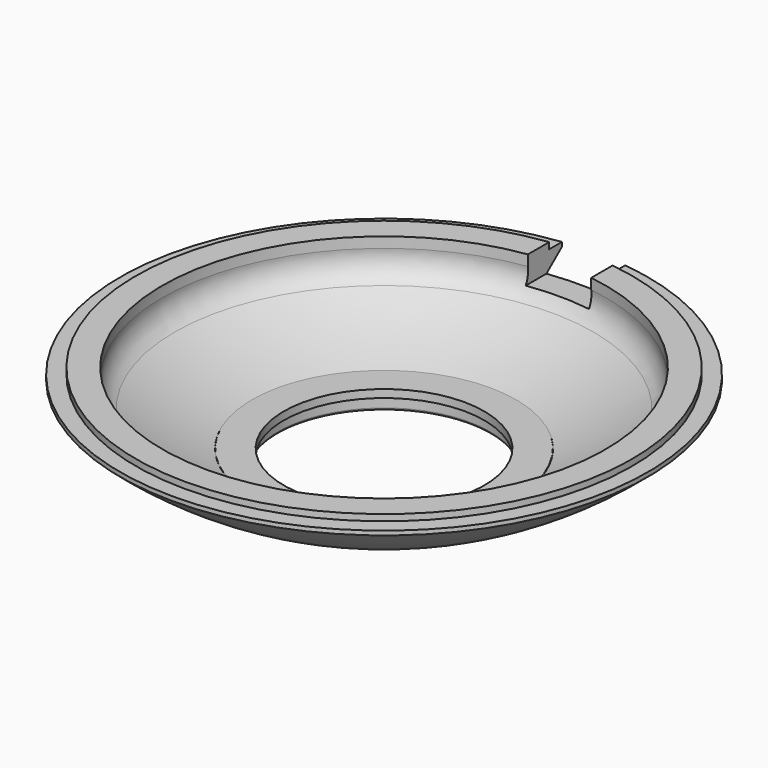
from build123d import *

# Parameters (mm, degrees)
F2_R     = 20
F3_DEPTH = 25
F4_R     = 2.5
F5_DEPTH = 25
F7_W     = 12
F7_H     = 6.6
F8_DEPTH = 60
F10_R    = 0.5
F9_W     = 6
F9_H     = 1.5


# Not quite as in the source:
# - a fillet or chamfer that OpenCascade refuses, or shapes differently, is made with other operations: its cross-section is extruded or revolved along the edge and cut away or added
# - a feature names something its author has since deleted; it is built from what else it names


with BuildPart() as f1:
    # F0 (on Right) → F1 (revolve)
    with BuildSketch(Plane.YZ):
        with BuildLine():
            ThreePointArc((0, -15), (-24.8151535342, -11.6208144071), (-47, 0))
            Line((-47, 0), (-42, 0))
            Line((-42, 0), (-42, 2))
            Line((-42, 2), (-47, 2))
            Line((-47, 2), (-47, 0.8))
            Line((-47, 0.8), (-50, 0.8))
            Line((-50, 0.8), (-50, 0))
            ThreePointArc((-50, 0), (-26.7070061906, -13.7416838627), (0, -18))
            Line((0, -18), (0, -15))
        make_face()
    revolve(axis=Axis((0, 0, -9), (0, 0, -1)))

    # F2 (on Top) → F3 (cut)
    with BuildSketch(Plane.XY):
        Circle(F2_R)
    extrude(amount=-F3_DEPTH, mode=Mode.SUBTRACT)

    # F4 (on Top) → F5 (cut)
    with BuildSketch(Plane.XY):
        with Locations((0, -26)):
            Circle(F4_R)
        with Locations((-22.5166604984, 13)):
            Circle(F4_R)
        with Locations((22.5166604984, 13)):
            Circle(F4_R)
    extrude(amount=F5_DEPTH, mode=Mode.SUBTRACT)

    # F6: fillet of radius 5 on 1 edges, made by hand

    # F6_s1 → F6_t2 (revolve)
    with BuildSketch(Plane.YZ):
        with BuildLine():
            ThreePointArc((-39.5886862508, -5.0098655294), (-41.5550423226, -2.8709998558), (-42.0003960381, 5.61589e-05))
            Line((-42.0003960381, 5.61589e-05), (-42.4955021036, 0.0702630102))
            ThreePointArc((-42.4955021036, 0.0702630102), (-44.5001980191, 0.5000590146), (-47, 0.5000590146))
            Line((-47, 0.5000590146), (-47.3050550292, -0.3962328195))
            ThreePointArc((-47.3050550292, -0.3962328195), (-43.6515985166, -3.0334873639), (-39.8426213376, -5.4406508469))
            Line((-39.8426213376, -5.4406508469), (-39.5886862508, -5.0098655294))
        make_face()
    revolve(axis=Axis((0, 0, 0), (0, 0, -1)))

    # F7 (on Front) → F8 (cut)
    with BuildSketch(Plane.XZ):
        with Locations((0, 0.3)):
            Rectangle(F7_W, F7_H)
    extrude(amount=-F8_DEPTH, mode=Mode.SUBTRACT)

    # F10
    f10_edges = [f1.edges().sort_by_distance(p)[0] for p in [
        (-14.142136, 14.142136, -15.795876),
        (14.142136, -14.142136, -15.795876),
    ]]
    fillet(f10_edges, radius=F10_R)

    # F9 (on Right) → F11 (revolve)
    with BuildSketch(Plane.YZ):
        with Locations((22, -12.25)):
            Rectangle(F9_W, F9_H)
    revolve(axis=Axis((0, 0, -5.7836989872), (0, 0, -1)))


solid = f1.part
